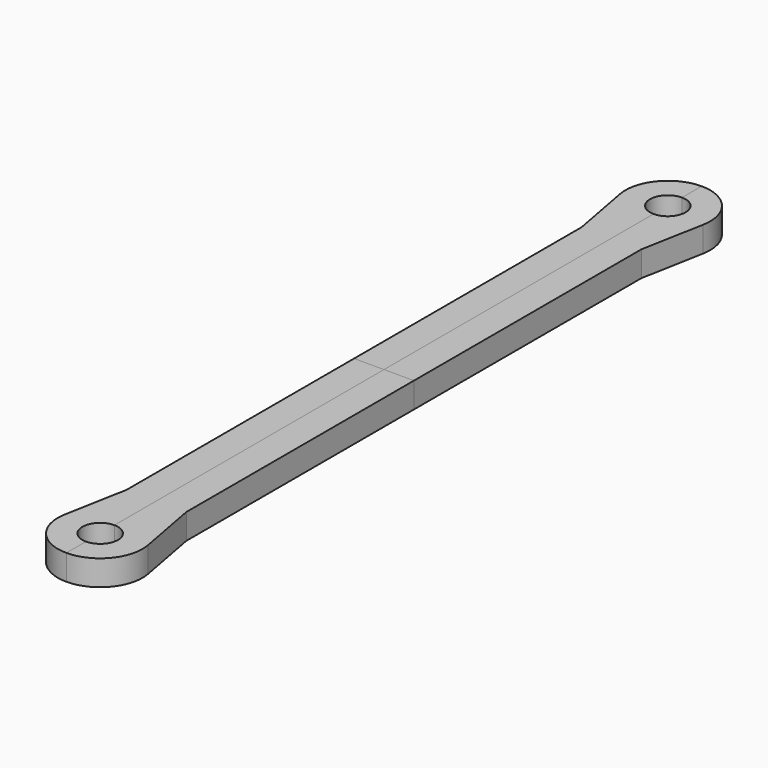
from build123d import *
from build123d import SkipClean  # not in build123d's __all__

# Parameters (mm, degrees)
F1_DEPTH = 2.8575


with BuildPart() as f1:
    # F0 (on Top) → F1 (new body, symmetric)
    with BuildSketch(Plane.XY):
        with BuildLine():
            ThreePointArc((0, -75.7864124179), (4, -79.7864124179), (0, -83.7864124179))
            Line((0, -83.7864124179), (0, -89.3016444676))
            ThreePointArc((0, -89.3016444676), (7.3191604153, -85.8666699597), (9.3539243357, -78.0417805136))
            Line((9.3539243357, -78.0417805136), (6.731, -63.9788508415))
            Line((6.731, -63.9788508415), (6.731, 0))
            Line((6.731, 0), (0, 0))
            Line((0, 0), (0, -75.7864124179))
        make_face()
    extrude(amount=F1_DEPTH, both=True)

    # F2: F1 across plane


with BuildPart() as f1_1:
    add(f1.part, clean=False)
    with SkipClean():  # cleaning this boolean's faces spoils the solid; the shape is the same uncleaned
        add(f1.part.mirror(Plane.YZ), clean=False)

    # F3: F1 across plane


with BuildPart() as f1_2:
    add(f1_1.part, clean=False)
    add(f1_1.part.mirror(Plane.XZ), clean=False)


solid = f1_2.part
